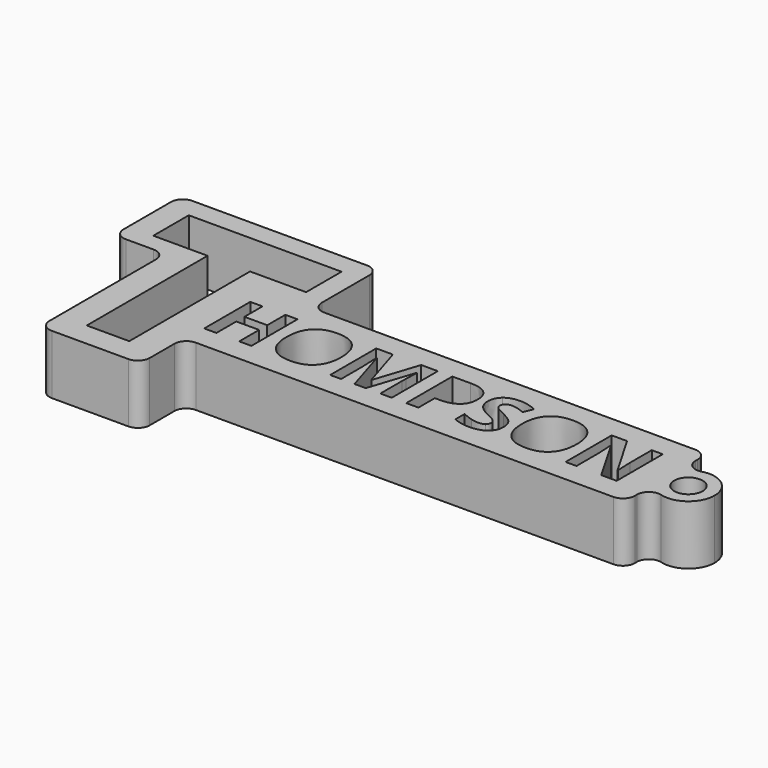
from build123d import *

# Parameters (mm, degrees)
F0_R     = 6.0091797901
F1_DEPTH = 25
F2_R     = 5


# Not quite as in the source:
# - a feature names something its author has since deleted; it is built from what else it names


with BuildPart() as f1:
    # F0 (on Top) → F1 (new body)
    with BuildSketch(Plane.XY):
        with BuildLine():
            Line((-20.1136302203, 0), (-20.1136302203, -57.1685433388))
            Line((-20.1136302203, -57.1685433388), (22.2150571644, -57.1685433388))
            Line((22.2150571644, -57.1685433388), (22.2150571644, -34.1469403356))
            Line((22.2150571644, -34.1469403356), (208.3863466978, -34.1469403356))
            Line((208.3863466978, -34.1469403356), (208.3863466978, -18.4070311298))
            ThreePointArc((208.3863466978, -18.4070311298), (206.7049342576, -12.5487698242), (208.3863466978, -6.6905085186))
            Line((208.3863466978, -6.6905085186), (208.3863466978, 9.0494006872))
            Line((208.3863466978, 9.0494006872), (41.8305061758, 9.0494006872))
            Line((41.8305061758, 9.0494006872), (41.8305061758, 44.1170223057))
            Line((41.8305061758, 44.1170223057), (-41.8593846262, 44.1170223057))
            Line((-41.8593846262, 44.1170223057), (-41.8593846262, 9.0494006872))
            Line((-41.8593846262, 9.0494006872), (-20.1136302203, 9.0494006872))
            Line((-20.1136302203, 9.0494006872), (-20.1136302203, 0))
        make_face()
        Polygon((42.9636666025, -0.2074100812), (42.9636666025, -24.5062988251), (37.8262784373, -24.5062988251), (37.8262784373, -14.0187942064), (28.2056415939, -14.0187942064), (28.2056415939, -24.5062988251), (23.0522988071, -24.5062988251), (23.0522988071, -0.2074100812), (28.2056415939, -0.2074100812), (28.2056415939, -9.7323191949), (37.8262784373, -9.7323191949), (37.8262784373, -0.2074100812), align=None, mode=Mode.SUBTRACT)
        with BuildLine():
            add(Edge.make_bspline(
                [(68.1826051938, -3.0499918351), (71.1501648172, -6.2754845082), (71.1501648172, -12.3222861063)],
                knots=[0, 0, 0, 1, 1, 1], degree=2))
            add(Edge.make_bspline(
                [(71.1501648172, -12.3222861063), (71.1501648172, -18.35845129), (68.1586732614, -21.5998985847)],
                knots=[0, 0, 0, 1, 1, 1], degree=2))
            add(Edge.make_bspline(
                [(68.1586732614, -21.5998985847), (65.1671817056, -24.8413458794), (59.5830641347, -24.8413458794)],
                knots=[0, 0, 0, 1, 1, 1], degree=2))
            add(Edge.make_bspline(
                [(59.5830641347, -24.8413458794), (53.9989465639, -24.8413458794), (51.0074550081, -21.5998985847)],
                knots=[0, 0, 0, 1, 1, 1], degree=2))
            add(Edge.make_bspline(
                [(51.0074550081, -21.5998985847), (48.0159634523, -18.35845129), (48.0159634523, -12.290376863)],
                knots=[0, 0, 0, 1, 1, 1], degree=2))
            add(Edge.make_bspline(
                [(48.0159634523, -12.290376863), (48.0159634523, -6.2223024361), (51.0154323189, -3.0234007991)],
                knots=[0, 0, 0, 1, 1, 1], degree=2))
            add(Edge.make_bspline(
                [(51.0154323189, -3.0234007991), (54.0149011855, 0.1755008379), (59.614973378, 0.1755008379)],
                knots=[0, 0, 0, 1, 1, 1], degree=2))
            add(Edge.make_bspline(
                [(59.614973378, 0.1755008379), (65.2150455705, 0.1755008379), (68.1826051938, -3.0499918351)],
                knots=[0, 0, 0, 1, 1, 1], degree=2))
        make_face(mode=Mode.SUBTRACT)
        with BuildLine():
            Line((91.1944877929, -24.5062988251), (86.4719197901, -24.5062988251))
            Line((86.4719197901, -24.5062988251), (80.6218918588, -5.4458441834))
            Line((80.6218918588, -5.4458441834), (80.4729820569, -5.4458441834))
            add(Edge.make_bspline(
                [(80.4729820569, -5.4458441834), (80.7920744895, -11.2586446642), (80.7920744895, -13.2051085032)],
                knots=[0, 0, 0, 1, 1, 1], degree=2))
            Line((80.7920744895, -13.2051085032), (80.7920744895, -24.5062988251))
            Line((80.7920744895, -24.5062988251), (76.1865070453, -24.5062988251))
            Line((76.1865070453, -24.5062988251), (76.1865070453, -0.2074100812))
            Line((76.1865070453, -0.2074100812), (83.2012223558, -0.2074100812))
            Line((83.2012223558, -0.2074100812), (88.9502043501, -18.7892260741))
            Line((88.9502043501, -18.7892260741), (89.0512502871, -18.7892260741))
            Line((89.0512502871, -18.7892260741), (95.1512339573, -0.2074100812))
            Line((95.1512339573, -0.2074100812), (102.1606310605, -0.2074100812))
            Line((102.1606310605, -0.2074100812), (102.1606310605, -24.5062988251))
            Line((102.1606310605, -24.5062988251), (97.3582899496, -24.5062988251))
            Line((97.3582899496, -24.5062988251), (97.3582899496, -13.0030166292))
            add(Edge.make_bspline(
                [(97.3582899496, -13.0030166292), (97.3582899496, -12.189330926), (97.3848809857, -11.125689484)],
                knots=[0, 0, 0, 1, 1, 1], degree=2))
            add(Edge.make_bspline(
                [(97.3848809857, -11.125689484), (97.4114720217, -10.0620480419), (97.6082456885, -5.4777534266)],
                knots=[0, 0, 0, 1, 1, 1], degree=2))
            Line((97.6082456885, -5.4777534266), (97.4593358866, -5.4777534266))
            Line((97.4593358866, -5.4777534266), (91.1944877929, -24.5062988251))
        make_face(mode=Mode.SUBTRACT)
        with BuildLine():
            add(Edge.make_bspline(
                [(122.7607066897, -2.1113282625), (125.0608313082, -4.0152464438), (125.0608313082, -7.7858553559)],
                knots=[0, 0, 0, 1, 1, 1], degree=2))
            add(Edge.make_bspline(
                [(125.0608313082, -7.7858553559), (125.0608313082, -11.7106922771), (122.6091377842, -13.7874521927)],
                knots=[0, 0, 0, 1, 1, 1], degree=2))
            add(Edge.make_bspline(
                [(122.6091377842, -13.7874521927), (120.1574442603, -15.8642121084), (115.6369681315, -15.8642121084)],
                knots=[0, 0, 0, 1, 1, 1], degree=2))
            Line((115.6369681315, -15.8642121084), (113.4299121392, -15.8642121084))
            Line((113.4299121392, -15.8642121084), (113.4299121392, -24.5062988251))
            Line((113.4299121392, -24.5062988251), (108.2765693524, -24.5062988251))
            Line((108.2765693524, -24.5062988251), (108.2765693524, -0.2074100812))
            Line((108.2765693524, -0.2074100812), (116.0358336723, -0.2074100812))
            add(Edge.make_bspline(
                [(116.0358336723, -0.2074100812), (120.4605820712, -0.2074100812), (122.7607066897, -2.1113282625)],
                knots=[0, 0, 0, 1, 1, 1], degree=2))
        make_face(mode=Mode.SUBTRACT)
        with BuildLine():
            add(Edge.make_bspline(
                [(142.7305747645, -13.7449065351), (143.9936489769, -15.3802552522), (143.9936489769, -17.7574938753)],
                knots=[0, 0, 0, 1, 1, 1], degree=2))
            add(Edge.make_bspline(
                [(143.9936489769, -17.7574938753), (143.9936489769, -21.0494641384), (141.6243876647, -22.9454050089)],
                knots=[0, 0, 0, 1, 1, 1], degree=2))
            add(Edge.make_bspline(
                [(141.6243876647, -22.9454050089), (139.2551263525, -24.8413458794), (135.0377880347, -24.8413458794)],
                knots=[0, 0, 0, 1, 1, 1], degree=2))
            add(Edge.make_bspline(
                [(135.0377880347, -24.8413458794), (131.1448603568, -24.8413458794), (128.1560279046, -23.3735206893)],
                knots=[0, 0, 0, 1, 1, 1], degree=2))
            Line((128.1560279046, -23.3735206893), (128.1560279046, -18.5871342001))
            add(Edge.make_bspline(
                [(128.1560279046, -18.5871342001), (130.6130396357, -19.6880030926), (132.3175250466, -20.1347324983)],
                knots=[0, 0, 0, 1, 1, 1], degree=2))
            add(Edge.make_bspline(
                [(132.3175250466, -20.1347324983), (134.0220104576, -20.5814619039), (135.4366535755, -20.5814619039)],
                knots=[0, 0, 0, 1, 1, 1], degree=2))
            add(Edge.make_bspline(
                [(135.4366535755, -20.5814619039), (137.1278434684, -20.5814619039), (138.0345977977, -19.9352997279)],
                knots=[0, 0, 0, 1, 1, 1], degree=2))
            add(Edge.make_bspline(
                [(138.0345977977, -19.9352997279), (138.9413521271, -19.2891375518), (138.9413521271, -18.0074496141)],
                knots=[0, 0, 0, 1, 1, 1], degree=2))
            add(Edge.make_bspline(
                [(138.9413521271, -18.0074496141), (138.9413521271, -17.294809848), (138.5424865863, -16.7363980909)],
                knots=[0, 0, 0, 1, 1, 1], degree=2))
            add(Edge.make_bspline(
                [(138.5424865863, -16.7363980909), (138.1436210456, -16.1779863338), (137.3698218965, -15.664779338)],
                knots=[0, 0, 0, 1, 1, 1], degree=2))
            add(Edge.make_bspline(
                [(137.3698218965, -15.664779338), (136.5960227474, -15.1515723422), (134.2187841243, -14.0187942064)],
                knots=[0, 0, 0, 1, 1, 1], degree=2))
            add(Edge.make_bspline(
                [(134.2187841243, -14.0187942064), (131.9957735104, -12.971107386), (130.8816090999, -12.0085118809)],
                knots=[0, 0, 0, 1, 1, 1], degree=2))
            add(Edge.make_bspline(
                [(130.8816090999, -12.0085118809), (129.7674446893, -11.0459163758), (129.102668788, -9.7642284381)],
                knots=[0, 0, 0, 1, 1, 1], degree=2))
            add(Edge.make_bspline(
                [(129.102668788, -9.7642284381), (128.4378928867, -8.4825405005), (128.4378928867, -6.7753959859)],
                knots=[0, 0, 0, 1, 1, 1], degree=2))
            add(Edge.make_bspline(
                [(128.4378928867, -6.7753959859), (128.4378928867, -3.5472442093), (130.6236760502, -1.7044854109)],
                knots=[0, 0, 0, 1, 1, 1], degree=2))
            add(Edge.make_bspline(
                [(130.6236760502, -1.7044854109), (132.8094592136, 0.1382733875), (136.6651594411, 0.1382733875)],
                knots=[0, 0, 0, 1, 1, 1], degree=2))
            add(Edge.make_bspline(
                [(136.6651594411, 0.1382733875), (138.558441208, 0.1382733875), (140.2788812405, -0.3084560182)],
                knots=[0, 0, 0, 1, 1, 1], degree=2))
            add(Edge.make_bspline(
                [(140.2788812405, -0.3084560182), (141.999321273, -0.7551854239), (143.8766484183, -1.568871127)],
                knots=[0, 0, 0, 1, 1, 1], degree=2))
            Line((143.8766484183, -1.568871127), (142.2173677687, -5.5787993636))
            add(Edge.make_bspline(
                [(142.2173677687, -5.5787993636), (140.2709039297, -4.7810682821), (138.9998524064, -4.4646349531)],
                knots=[0, 0, 0, 1, 1, 1], degree=2))
            add(Edge.make_bspline(
                [(138.9998524064, -4.4646349531), (137.7288008831, -4.148201624), (136.5002950176, -4.148201624)],
                knots=[0, 0, 0, 1, 1, 1], degree=2))
            add(Edge.make_bspline(
                [(136.5002950176, -4.148201624), (135.0377880347, -4.148201624), (134.2560115748, -4.828932147)],
                knots=[0, 0, 0, 1, 1, 1], degree=2))
            add(Edge.make_bspline(
                [(134.2560115748, -4.828932147), (133.4742351149, -5.5096626699), (133.4742351149, -6.6052133552)],
                knots=[0, 0, 0, 1, 1, 1], degree=2))
            add(Edge.make_bspline(
                [(133.4742351149, -6.6052133552), (133.4742351149, -7.2859438781), (133.7906684439, -7.7938326667)],
                knots=[0, 0, 0, 1, 1, 1], degree=2))
            add(Edge.make_bspline(
                [(133.7906684439, -7.7938326667), (134.1071017729, -8.3017214553), (134.7958096067, -8.775041897)],
                knots=[0, 0, 0, 1, 1, 1], degree=2))
            add(Edge.make_bspline(
                [(134.7958096067, -8.775041897), (135.4845174404, -9.2483623387), (138.0585297302, -10.4768682043)],
                knots=[0, 0, 0, 1, 1, 1], degree=2))
            add(Edge.make_bspline(
                [(138.0585297302, -10.4768682043), (141.467500552, -12.1095578179), (142.7305747645, -13.7449065351)],
                knots=[0, 0, 0, 1, 1, 1], degree=2))
        make_face(mode=Mode.SUBTRACT)
        with BuildLine():
            add(Edge.make_bspline(
                [(167.4841702249, -3.0499918351), (170.4517298482, -6.2754845082), (170.4517298482, -12.3222861063)],
                knots=[0, 0, 0, 1, 1, 1], degree=2))
            add(Edge.make_bspline(
                [(170.4517298482, -12.3222861063), (170.4517298482, -18.35845129), (167.4602382924, -21.5998985847)],
                knots=[0, 0, 0, 1, 1, 1], degree=2))
            add(Edge.make_bspline(
                [(167.4602382924, -21.5998985847), (164.4687467366, -24.8413458794), (158.8846291658, -24.8413458794)],
                knots=[0, 0, 0, 1, 1, 1], degree=2))
            add(Edge.make_bspline(
                [(158.8846291658, -24.8413458794), (153.300511595, -24.8413458794), (150.3090200392, -21.5998985847)],
                knots=[0, 0, 0, 1, 1, 1], degree=2))
            add(Edge.make_bspline(
                [(150.3090200392, -21.5998985847), (147.3175284834, -18.35845129), (147.3175284834, -12.290376863)],
                knots=[0, 0, 0, 1, 1, 1], degree=2))
            add(Edge.make_bspline(
                [(147.3175284834, -12.290376863), (147.3175284834, -6.2223024361), (150.31699735, -3.0234007991)],
                knots=[0, 0, 0, 1, 1, 1], degree=2))
            add(Edge.make_bspline(
                [(150.31699735, -3.0234007991), (153.3164662166, 0.1755008379), (158.9165384091, 0.1755008379)],
                knots=[0, 0, 0, 1, 1, 1], degree=2))
            add(Edge.make_bspline(
                [(158.9165384091, 0.1755008379), (164.5166106015, 0.1755008379), (167.4841702249, -3.0499918351)],
                knots=[0, 0, 0, 1, 1, 1], degree=2))
        make_face(mode=Mode.SUBTRACT)
        with BuildLine():
            Line((197.0427658998, -0.2074100812), (197.0427658998, -24.5062988251))
            Line((197.0427658998, -24.5062988251), (190.4960528239, -24.5062988251))
            Line((190.4960528239, -24.5062988251), (179.9234568898, -6.1265747063))
            Line((179.9234568898, -6.1265747063), (179.7745470879, -6.1265747063))
            add(Edge.make_bspline(
                [(179.7745470879, -6.1265747063), (180.0936395205, -10.9927343037), (180.0936395205, -13.072153323)],
                knots=[0, 0, 0, 1, 1, 1], degree=2))
            Line((180.0936395205, -13.072153323), (180.0936395205, -24.5062988251))
            Line((180.0936395205, -24.5062988251), (175.4880720764, -24.5062988251))
            Line((175.4880720764, -24.5062988251), (175.4880720764, -0.2074100812))
            Line((175.4880720764, -0.2074100812), (181.9869212874, -0.2074100812))
            Line((181.9869212874, -0.2074100812), (192.5382443927, -18.4063151549))
            Line((192.5382443927, -18.4063151549), (192.6552449513, -18.4063151549))
            add(Edge.make_bspline(
                [(192.6552449513, -18.4063151549), (192.4052892124, -13.6677925305), (192.4052892124, -11.7106922771)],
                knots=[0, 0, 0, 1, 1, 1], degree=2))
            Line((192.4052892124, -11.7106922771), (192.4052892124, -0.2074100812))
            Line((192.4052892124, -0.2074100812), (197.0427658998, -0.2074100812))
        make_face(mode=Mode.SUBTRACT)
        Polygon((-31.3512943685, 35.36279127), (33.0937728286, 35.36279127), (33.0937728286, 16.6775323451), (9.4512049109, 16.6775323451), (9.4512049109, -47.0048710704), (-8.4713893011, -47.0048710704), (-8.4713893011, 16.6775323451), (-31.3512943685, 16.6775323451), align=None, mode=Mode.SUBTRACT)
        with BuildLine():
            Line((208.3863466978, -6.6905085186), (208.3863466978, -18.4070311298))
            ThreePointArc((208.3863466978, -18.4070311298), (220.798506794, -23.1662802691), (228.7972968634, -12.5487698242))
            ThreePointArc((228.7972968634, -12.5487698242), (220.798506794, -1.9312593793), (208.3863466978, -6.6905085186))
        make_face()
        with Locations((217.7511155605, -12.5487698242)):
            Circle(F0_R, mode=Mode.SUBTRACT)
        with BuildLine():
            ThreePointArc((208.3863466978, -6.6905085186), (206.7049342576, -12.5487698242), (208.3863466978, -18.4070311298))
            Line((208.3863466978, -18.4070311298), (208.3863466978, -6.6905085186))
        make_face()
    extrude(amount=F1_DEPTH)

    # F2
    f2_edges = [f1.edges().sort_by_distance(p)[0] for p in [
        (208.386347, -6.690509, 12.5),
        (208.386347, -18.407031, 12.5),
        (22.215057, -34.14694, 12.5),
        (22.215057, -57.168543, 12.5),
        (-20.11363, -57.168543, 12.5),
        (208.386347, -34.14694, 12.5),
        (-20.11363, 9.049401, 12.5),
        (-41.859385, 9.049401, 12.5),
        (-41.859385, 44.117022, 12.5),
        (41.830506, 44.117022, 12.5),
        (41.830506, 9.049401, 12.5),
        (208.386347, 9.049401, 12.5),
    ]]
    fillet(f2_edges, radius=F2_R)


solid = f1.part
